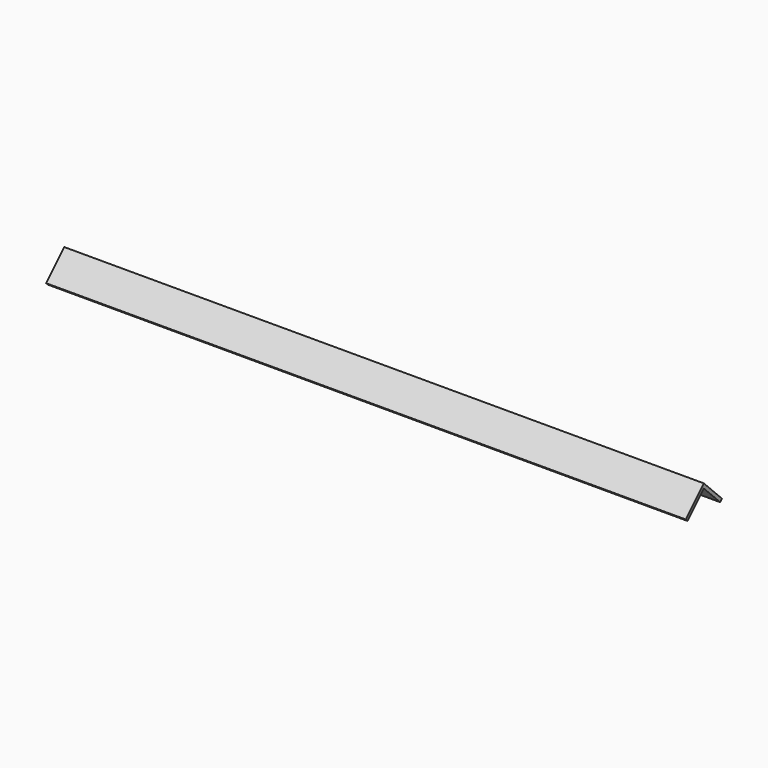
from build123d import *

# Parameters (mm, degrees)
F1_E0_W  = 50
F1_E0_H  = 1000
F2_DEPTH = 5
F1_E1_W  = 50
F1_E1_H  = 1000
F3_DEPTH = 5


with BuildPart() as f2:
    # F1_E0 (on explicit) → F2 (new body)
    with BuildSketch(Plane(origin=(0, -35.3553390593, 0), x_dir=(0, 0.7071067812, 0.7071067812), z_dir=(0, 0.7071067812, -0.7071067812))):
        with Locations((25, 500)):
            Rectangle(F1_E0_W, F1_E0_H)
    extrude(amount=F2_DEPTH)

    # F1_E1 (on explicit) → F3 (join)
    with BuildSketch(Plane(origin=(0, 0, 35.3553390593), x_dir=(0, 0.7071067812, -0.7071067812), z_dir=(0, -0.7071067812, -0.7071067812))):
        with Locations((25, 500)):
            Rectangle(F1_E1_W, F1_E1_H)
    extrude(amount=F3_DEPTH)


solid = f2.part
